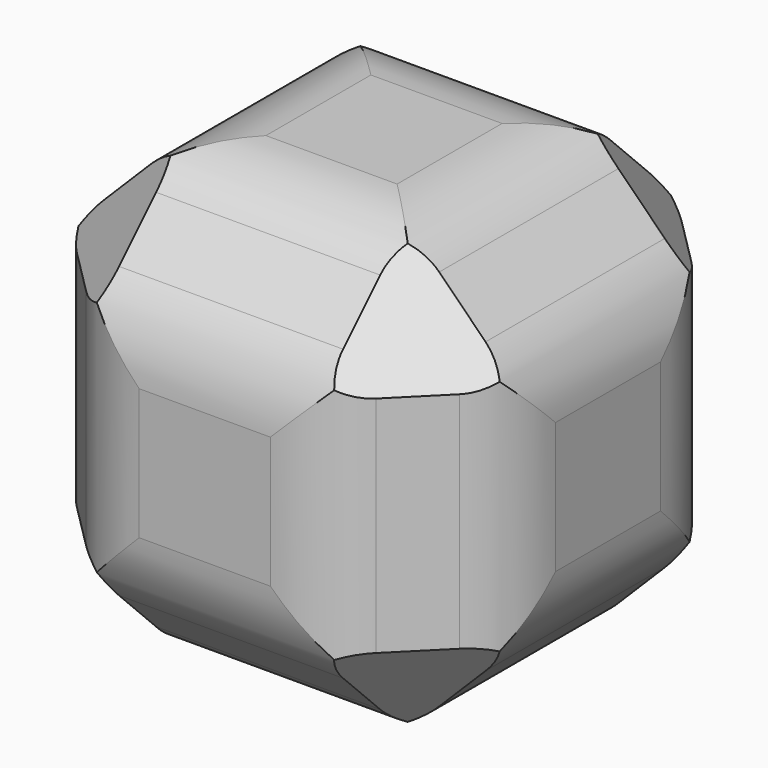
from build123d import *

# Parameters (mm, degrees)
F0_W        = 20
F0_H        = 20
F1_DEPTH    = 20
F2_SIZE     = 5
F3_T1_DEPTH = 20.3553390593
F3_T3_DEPTH = 20.3553390593
F3_T5_DEPTH = 20.3553390593


# Not quite as in the source:
# - a fillet or chamfer that OpenCascade refuses, or shapes differently, is made with other operations: its cross-section is extruded or revolved along the edge and cut away or added


with BuildPart() as f1:
    # F0 (on Top) → F1 (new body)
    with BuildSketch(Plane.XY):
        with Locations((8.6001078598, -0.1764608825)):
            Rectangle(F0_W, F0_H)
    extrude(amount=F1_DEPTH)

    # F2
    f2_edges = [f1.edges().sort_by_distance(p)[0] for p in [
        (8.600108, -10.176461, 20),
        (18.600108, -0.176461, 20),
        (8.600108, 9.823539, 20),
        (-1.399892, -0.176461, 20),
        (-1.399892, -0.176461, 0),
        (8.600108, 9.823539, 0),
        (18.600108, -0.176461, 0),
        (8.600108, -10.176461, 0),
        (-1.399892, 9.823539, 10),
        (18.600108, 9.823539, 10),
        (18.600108, -10.176461, 10),
        (-1.399892, -10.176461, 10),
    ]]
    chamfer(f2_edges, length=F2_SIZE)

    # F3: fillet of radius 5 on 24 edges, made by hand

    # F3_s2 → F3_t1 (cut)
    with BuildSketch(Plane.XZ.offset(-10.0012086472)):
        with BuildLine():
            ThreePointArc((11.529040048, 0), (13.4424572098, 0.3806023374), (15.0645739539, 1.4644660941))
            Line((15.0645739539, 1.4644660941), (13.6001078598, 0))
            Line((13.6001078598, 0), (11.529040048, 0))
        make_face()
        with BuildLine():
            ThreePointArc((18.6001078598, 7.0710678119), (18.2195055224, 5.15765065), (17.1356417658, 3.5355339059))
            Line((17.1356417658, 3.5355339059), (18.6001078598, 5))
            Line((18.6001078598, 5), (18.6001078598, 7.0710678119))
        make_face()
        with BuildLine():
            ThreePointArc((18.6001078598, 12.9289321881), (18.2195055224, 14.84234935), (17.1356417658, 16.4644660941))
            Line((17.1356417658, 16.4644660941), (18.6001078598, 15))
            Line((18.6001078598, 15), (18.6001078598, 12.9289321881))
        make_face()
        with BuildLine():
            ThreePointArc((11.529040048, 20), (13.4424572098, 19.6193976626), (15.0645739539, 18.5355339059))
            Line((15.0645739539, 18.5355339059), (13.6001078598, 20))
            Line((13.6001078598, 20), (11.529040048, 20))
        make_face()
        with BuildLine():
            ThreePointArc((5.6711756717, 20), (3.7577585099, 19.6193976626), (2.1356417658, 18.5355339059))
            Line((2.1356417658, 18.5355339059), (3.6001078598, 20))
            Line((3.6001078598, 20), (5.6711756717, 20))
        make_face()
        with BuildLine():
            ThreePointArc((-1.3998921402, 12.9289321881), (-1.0192898027, 14.84234935), (0.0645739539, 16.4644660941))
            Line((0.0645739539, 16.4644660941), (-1.3998921402, 15))
            Line((-1.3998921402, 15), (-1.3998921402, 12.9289321881))
        make_face()
        with BuildLine():
            ThreePointArc((-1.3998921402, 7.0710678119), (-1.0192898027, 5.15765065), (0.0645739539, 3.5355339059))
            Line((0.0645739539, 3.5355339059), (-1.3998921402, 5))
            Line((-1.3998921402, 5), (-1.3998921402, 7.0710678119))
        make_face()
        with BuildLine():
            ThreePointArc((5.6711756717, 0), (3.7577585099, 0.3806023374), (2.1356417658, 1.4644660941))
            Line((2.1356417658, 1.4644660941), (3.6001078598, 0))
            Line((3.6001078598, 0), (5.6711756717, 0))
        make_face()
    extrude(amount=F3_T1_DEPTH, mode=Mode.SUBTRACT)

    # F3_s4 → F3_t3 (cut)
    with BuildSketch(Plane.YZ.offset(-1.5775616698)):
        with BuildLine():
            ThreePointArc((9.8235391175, 7.0710678119), (9.4429367801, 5.15765065), (8.3590730234, 3.5355339059))
            Line((8.3590730234, 3.5355339059), (9.8235391175, 5))
            Line((9.8235391175, 5), (9.8235391175, 7.0710678119))
        make_face()
        with BuildLine():
            ThreePointArc((9.8235391175, 12.9289321881), (9.4429367801, 14.84234935), (8.3590730234, 16.4644660941))
            Line((8.3590730234, 16.4644660941), (9.8235391175, 15))
            Line((9.8235391175, 15), (9.8235391175, 12.9289321881))
        make_face()
        with BuildLine():
            ThreePointArc((6.2880052116, 1.4644660941), (4.6658884675, 0.3806023374), (2.7524713056, 0))
            Line((2.7524713056, 0), (4.8235391175, 0))
            Line((4.8235391175, 0), (6.2880052116, 1.4644660941))
        make_face()
        with BuildLine():
            ThreePointArc((-3.1053930706, 0), (-5.0188102325, 0.3806023374), (-6.6409269766, 1.4644660941))
            Line((-6.6409269766, 1.4644660941), (-5.1764608825, 0))
            Line((-5.1764608825, 0), (-3.1053930706, 0))
        make_face()
        with BuildLine():
            ThreePointArc((-8.7119947884, 3.5355339059), (-9.795858545, 5.15765065), (-10.1764608825, 7.0710678119))
            Line((-10.1764608825, 7.0710678119), (-10.1764608825, 5))
            Line((-10.1764608825, 5), (-8.7119947884, 3.5355339059))
        make_face()
        with BuildLine():
            ThreePointArc((-8.7119947884, 16.4644660941), (-9.795858545, 14.84234935), (-10.1764608825, 12.9289321881))
            Line((-10.1764608825, 12.9289321881), (-10.1764608825, 15))
            Line((-10.1764608825, 15), (-8.7119947884, 16.4644660941))
        make_face()
        with BuildLine():
            ThreePointArc((-3.1053930706, 20), (-5.0188102325, 19.6193976626), (-6.6409269766, 18.5355339059))
            Line((-6.6409269766, 18.5355339059), (-5.1764608825, 20))
            Line((-5.1764608825, 20), (-3.1053930706, 20))
        make_face()
        with BuildLine():
            ThreePointArc((6.2880052116, 18.5355339059), (4.6658884675, 19.6193976626), (2.7524713056, 20))
            Line((2.7524713056, 20), (4.8235391175, 20))
            Line((4.8235391175, 20), (6.2880052116, 18.5355339059))
        make_face()
    extrude(amount=F3_T3_DEPTH, mode=Mode.SUBTRACT)

    # F3_s6 → F3_t5 (cut)
    with BuildSketch(Plane.XY.offset(-0.1776695297)):
        with BuildLine():
            ThreePointArc((0.0645739539, 6.2880052116), (-1.0192898027, 4.6658884675), (-1.3998921402, 2.7524713056))
            Line((-1.3998921402, 2.7524713056), (-1.3998921402, 4.8235391175))
            Line((-1.3998921402, 4.8235391175), (0.0645739539, 6.2880052116))
        make_face()
        with BuildLine():
            ThreePointArc((5.6711756717, 9.8235391175), (3.7577585099, 9.4429367801), (2.1356417658, 8.3590730234))
            Line((2.1356417658, 8.3590730234), (3.6001078598, 9.8235391175))
            Line((3.6001078598, 9.8235391175), (5.6711756717, 9.8235391175))
        make_face()
        with BuildLine():
            ThreePointArc((11.529040048, 9.8235391175), (13.4424572098, 9.4429367801), (15.0645739539, 8.3590730234))
            Line((15.0645739539, 8.3590730234), (13.6001078598, 9.8235391175))
            Line((13.6001078598, 9.8235391175), (11.529040048, 9.8235391175))
        make_face()
        with BuildLine():
            ThreePointArc((17.1356417658, 6.2880052116), (18.2195055224, 4.6658884675), (18.6001078598, 2.7524713056))
            Line((18.6001078598, 2.7524713056), (18.6001078598, 4.8235391175))
            Line((18.6001078598, 4.8235391175), (17.1356417658, 6.2880052116))
        make_face()
        with BuildLine():
            ThreePointArc((18.6001078598, -3.1053930706), (18.2195055224, -5.0188102325), (17.1356417658, -6.6409269766))
            Line((17.1356417658, -6.6409269766), (18.6001078598, -5.1764608825))
            Line((18.6001078598, -5.1764608825), (18.6001078598, -3.1053930706))
        make_face()
        with BuildLine():
            ThreePointArc((15.0645739539, -8.7119947884), (13.4424572098, -9.795858545), (11.529040048, -10.1764608825))
            Line((11.529040048, -10.1764608825), (13.6001078598, -10.1764608825))
            Line((13.6001078598, -10.1764608825), (15.0645739539, -8.7119947884))
        make_face()
        with BuildLine():
            ThreePointArc((2.1356417658, -8.7119947884), (3.7577585099, -9.795858545), (5.6711756717, -10.1764608825))
            Line((5.6711756717, -10.1764608825), (3.6001078598, -10.1764608825))
            Line((3.6001078598, -10.1764608825), (2.1356417658, -8.7119947884))
        make_face()
        with BuildLine():
            ThreePointArc((-1.3998921402, -3.1053930706), (-1.0192898027, -5.0188102325), (0.0645739539, -6.6409269766))
            Line((0.0645739539, -6.6409269766), (-1.3998921402, -5.1764608825))
            Line((-1.3998921402, -5.1764608825), (-1.3998921402, -3.1053930706))
        make_face()
    extrude(amount=F3_T5_DEPTH, mode=Mode.SUBTRACT)


solid = f1.part
